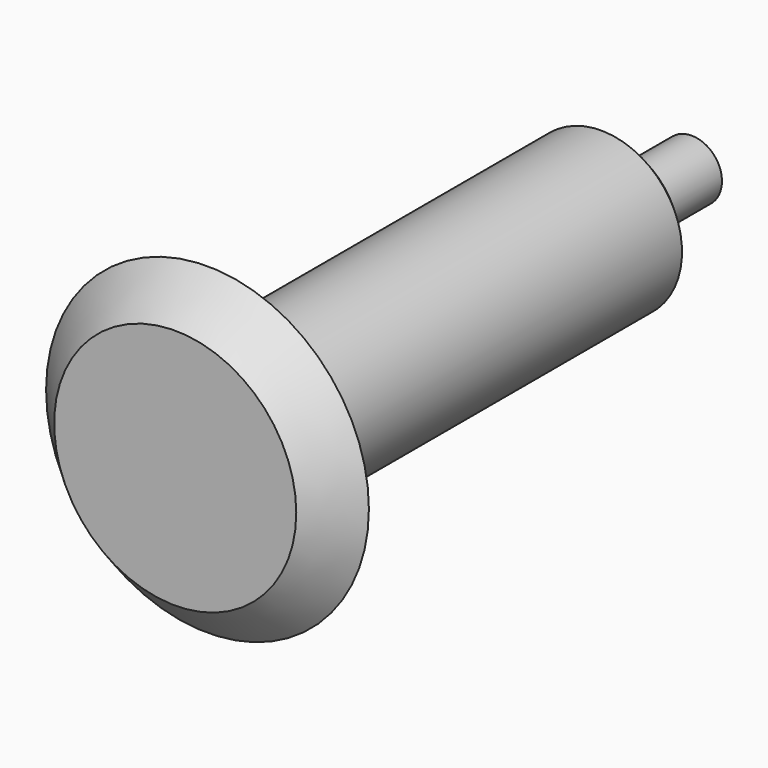
from build123d import *

# Parameters (mm, degrees)
F0_R      = 40
F1_DEPTH  = 10
F3_SIZE   = 9.99999
F2_R      = 30
F4_DEPTH  = 10
F5_SIZE   = 9.99999
F6_R      = 20
F7_DEPTH  = 115
F8_SIZE   = 3
F9_R      = 7.5
F10_DEPTH = 25


# Not quite as in the source:
# - a fillet or chamfer is up to 0.001 mm smaller than in the source, because OpenCascade refuses the exact size


with BuildPart() as f1:
    # F0 (on Front) → F1 (new body)
    with BuildSketch(Plane.XZ):
        Circle(F0_R)
    extrude(amount=F1_DEPTH)

    # F3 (size 10 in the source; OpenCascade refuses exactly that, so slightly less here)
    f3_edges = [f1.edges().sort_by_distance(p)[0] for p in [
        (-40, -10, 0),
    ]]
    chamfer(f3_edges, length=F3_SIZE)

    # F2 (on face) → F4 (join)
    with BuildSketch(Plane(origin=(0, 0, 0), x_dir=(-1, 0, 0), z_dir=(0, 1, 0))):
        Circle(F2_R)
    extrude(amount=F4_DEPTH)

    # F5 (size 10 in the source; OpenCascade refuses exactly that, so slightly less here)
    f5_edges = [f1.edges().sort_by_distance(p)[0] for p in [
        (30, 10, 0),
    ]]
    chamfer(f5_edges, length=F5_SIZE)

    # F6 (on face) → F7 (join)
    with BuildSketch(Plane(origin=(0, 10, 0), x_dir=(-1, 0, 0), z_dir=(0, 1, 0))):
        Circle(F6_R)
    extrude(amount=F7_DEPTH)

    # F8
    f8_edges = [f1.edges().sort_by_distance(p)[0] for p in [
        (20, 125, 0),
    ]]
    chamfer(f8_edges, length=F8_SIZE)

    # F9 (on face) → F10 (join)
    with BuildSketch(Plane(origin=(0, 125, 0), x_dir=(-1, 0, 0), z_dir=(0, 1, 0))):
        Circle(F9_R)
    extrude(amount=F10_DEPTH)


solid = f1.part
